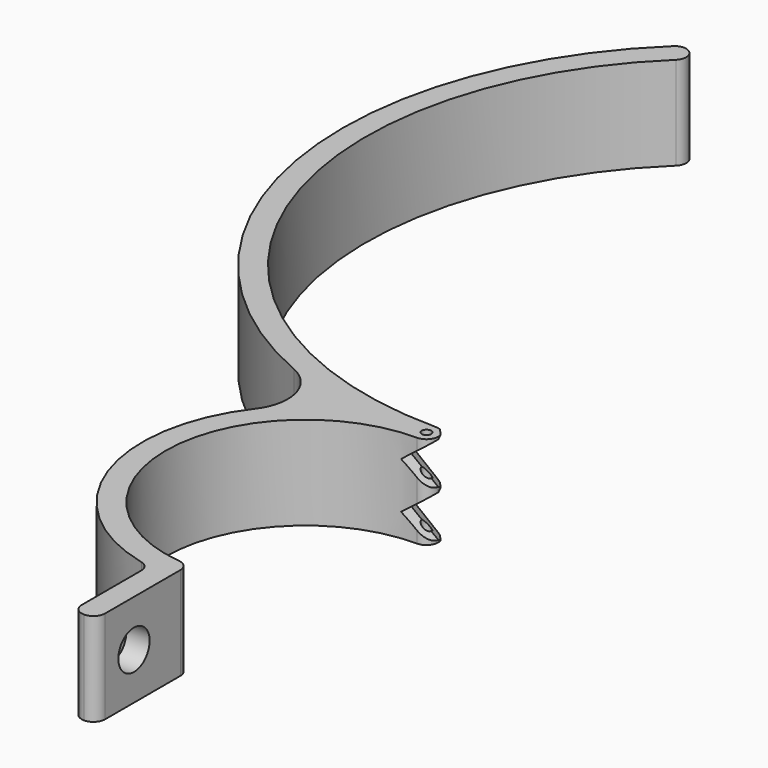
from build123d import *

# Parameters (mm, degrees)
F1_DEPTH       = 10
F2_W           = 45
F2_H           = 10
F3_DEPTH       = 10
F4_R           = 0.5
F5_DEPTH       = 10
F6_R           = 2.1
F7_DEPTH       = 2.5
F8_T1_DEPTH    = 10
F8_T3_DEPTH    = 43.0998702926
F9_T1_DEPTH    = 10
F9_T3_DEPTH    = 15.8191503542
F9_T5_DEPTH    = 16.25
F9_T7_DEPTH    = 36.3051320704
F11_DEPTH      = 5
F11_TAPER      = -30
F11_DEPTH_BACK = 5


# Not quite as in the source:
# - a fillet or chamfer that OpenCascade refuses, or shapes differently, is made with other operations: its cross-section is extruded or revolved along the edge and cut away or added


with BuildPart() as f1:
    # F0 (on Top) → F1 (new body)
    with BuildSketch(Plane.XY):
        with BuildLine():
            ThreePointArc((0, -1.25), (0.8838834765, -0.8838834765), (1.25, 0))
            ThreePointArc((1.25, 0), (0.8838834765, 0.8838834765), (0, 1.25))
            ThreePointArc((0, 1.25), (-1.25, 0), (0, -1.25))
        make_face()
        with BuildLine():
            ThreePointArc((0, -1.25), (-1.25, 0), (0, 1.25))
            ThreePointArc((0, 1.25), (-3.9258033341, 0.8039751431), (-7.6514917116, -0.5113636364))
            ThreePointArc((-7.6514917116, -0.5113636364), (-3.8435305739, -1.0649126927), (0, -1.25))
        make_face()
        with BuildLine():
            ThreePointArc((-7.6514917116, -0.5113636364), (-3.9258033341, 0.8039751431), (0, 1.25))
            ThreePointArc((0, 1.25), (-37.5, 38.75), (0, 76.25))
            Line((0, 76.25), (0, 78.75))
            ThreePointArc((0, 78.75), (-39.8149126927, 42.5935305739), (-7.6514917116, -0.5113636364))
        make_face()
        with BuildLine():
            ThreePointArc((-0.5, -31.2416643506), (-14.9979159429, -15.9999652609), (0, -1.25))
            ThreePointArc((0, -1.25), (-3.8435305739, -1.0649126927), (-7.6514917116, -0.5113636364))
            ThreePointArc((-7.6514917116, -0.5113636364), (-17.3284932243, -18.69403817), (-3, -33.4909396496))
            Line((-3, -33.4909396496), (-3, -31.2416643506))
            Line((-3, -31.2416643506), (-0.5, -31.2416643506))
        make_face()
        with BuildLine():
            Line((-0.5, -33.7428556845), (-0.5, -31.2416643506))
            Line((-0.5, -31.2416643506), (-3, -31.2416643506))
            Line((-3, -31.2416643506), (-3, -33.4909396496))
            ThreePointArc((-3, -33.4909396496), (-1.7545271221, -33.661824562), (-0.5, -33.7428556845))
        make_face()
        with BuildLine():
            ThreePointArc((-0.5, -33.7428556845), (-1.7545271221, -33.661824562), (-3, -33.4909396496))
            Line((-3, -33.4909396496), (-3, -43.7428556845))
            Line((-3, -43.7428556845), (-0.5, -43.7428556845))
            Line((-0.5, -43.7428556845), (-0.5, -33.7428556845))
        make_face()
    extrude(amount=F1_DEPTH)

    # F2 (on Top) → F3 (cut, through all)
    with BuildSketch(Plane.XY):
        with Locations((0, 73.75)):
            Rectangle(F2_W, F2_H)
    extrude(amount=F3_DEPTH, mode=Mode.SUBTRACT)

    # F4 (on face) → F5 (cut, through all)
    with BuildSketch(Plane.XY.offset(10)):
        Circle(F4_R)
    extrude(amount=-F5_DEPTH, mode=Mode.SUBTRACT)

    # F6 (on face) → F7 (cut, through all)
    with BuildSketch(Plane(origin=(-3, 0, 0), x_dir=(0, -1, 0), z_dir=(-1, 0, 0))):
        with Locations((38.6168976671, 5)):
            Circle(F6_R)
    extrude(amount=-F7_DEPTH, mode=Mode.SUBTRACT)

    # F8: fillet of radius 5 on 2 edges, made by hand

    # F8_s2 → F8_t1 (join)
    with BuildSketch(Plane.XY):
        with BuildLine():
            ThreePointArc((-13.8860405137, -5.5997474747), (-13.0142523991, -1.2990941124), (-15.8697605871, 2.0328282828))
            ThreePointArc((-15.8697605871, 2.0328282828), (-11.8292246388, 0.5391449396), (-7.6514917116, -0.5113636364))
            ThreePointArc((-7.6514917116, -0.5113636364), (-11.0652264374, -2.6923171637), (-13.8860405137, -5.5997474747))
        make_face()
    extrude(amount=F8_T1_DEPTH)

    # F8_s4 → F8_t3 (cut)
    with BuildSketch(Plane.XY.offset(-16.5499351463)):
        with BuildLine():
            ThreePointArc((-22.5, 68.75), (-25.2284691248, 68.9356152516), (-27.6464669917, 67.6580068991))
            ThreePointArc((-27.6464669917, 67.6580068991), (-25.1595214868, 69.8465991477), (-22.5, 71.8218913883))
            Line((-22.5, 71.8218913883), (-22.5, 68.75))
        make_face()
    extrude(amount=F8_T3_DEPTH, mode=Mode.SUBTRACT)

    # F9: fillet of radius 1.25 on 5 edges, made by hand

    # F9_s2 → F9_t1 (join)
    with BuildSketch(Plane.XY):
        with BuildLine():
            ThreePointArc((-3, -34.5119823677), (-3.2710549896, -33.73470078), (-3.9666666667, -33.2945168766))
            ThreePointArc((-3.9666666667, -33.2945168766), (-3.4847175764, -33.3995406181), (-3, -33.4909396496))
            Line((-3, -33.4909396496), (-3, -34.5119823677))
        make_face()
    extrude(amount=F9_T1_DEPTH)

    # F9_s4 → F9_t3 (cut)
    with BuildSketch(Plane.XY.offset(-2.9095751771)):
        with BuildLine():
            ThreePointArc((-1.6153846154, -31.1627640813), (-0.8197394906, -31.5705600619), (-0.5, -32.4054944214))
            Line((-0.5, -32.4054944214), (-0.5, -31.2416643506))
            ThreePointArc((-0.5, -31.2416643506), (-1.0584277637, -31.2126110913), (-1.6153846154, -31.1627640813))
        make_face()
    extrude(amount=F9_T3_DEPTH, mode=Mode.SUBTRACT)

    # F9_s6 → F9_t5 (cut)
    with BuildSketch(Plane.XY.offset(-3.125)):
        with BuildLine():
            ThreePointArc((-0.5, -42.4928556845), (-0.8661165235, -43.376739161), (-1.75, -43.7428556845))
            Line((-1.75, -43.7428556845), (-0.5, -43.7428556845))
            Line((-0.5, -43.7428556845), (-0.5, -42.4928556845))
        make_face()
        with BuildLine():
            ThreePointArc((-1.75, -43.7428556845), (-2.6338834765, -43.376739161), (-3, -42.4928556845))
            Line((-3, -42.4928556845), (-3, -43.7428556845))
            Line((-3, -43.7428556845), (-1.75, -43.7428556845))
        make_face()
    extrude(amount=F9_T5_DEPTH, mode=Mode.SUBTRACT)

    # F9_s8 → F9_t7 (cut)
    with BuildSketch(Plane.XY.offset(-13.1525660352)):
        with BuildLine():
            ThreePointArc((-25.9185526928, 65.8512661385), (-25.8791274069, 67.6185918599), (-27.6464530598, 67.658020223))
            ThreePointArc((-27.6464530598, 67.658020223), (-25.2284596959, 68.9356172522), (-22.5, 68.75))
            ThreePointArc((-22.5, 68.75), (-24.2526230688, 67.3517529932), (-25.9185526928, 65.8512661385))
        make_face()
    extrude(amount=F9_T7_DEPTH, mode=Mode.SUBTRACT)

    # F10 (on Front) → F11 (cut, two sides)
    with BuildSketch(Plane.XZ) as f11_sk:
        Polygon((1.5, 0.0747326796), (1.5, 4.9252673204), (-1.6606699079, 2.5), align=None)
        Polygon((1.5, 9.9252673204), (-1.6606699079, 7.5), (1.5, 5.0747326796), align=None)
    extrude(amount=-F11_DEPTH, taper=F11_TAPER, mode=Mode.SUBTRACT)
    extrude(f11_sk.sketch, amount=F11_DEPTH_BACK, mode=Mode.SUBTRACT)


solid = f1.part
